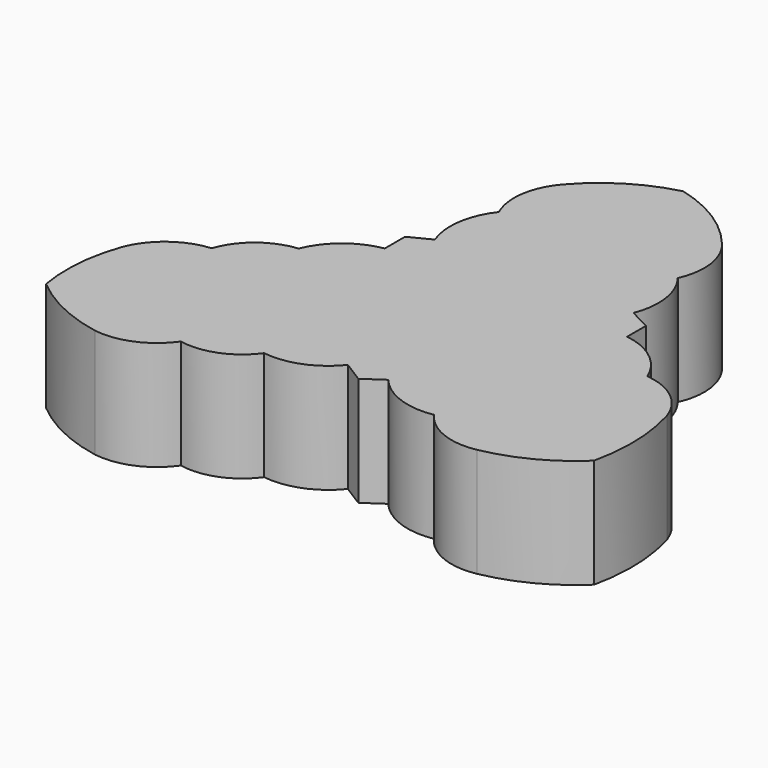
from build123d import *

# Parameters (mm, degrees)
F1_DEPTH = 11.1125


# Not quite as in the source:
# - a length typed as a fraction of an inch, garbled in the dataset ("3 / 203.2 mm" for 3/8 in), is restored


with BuildPart() as f1:
    # F0 (on Top) → F1 (new body)
    with BuildSketch(Plane.XY):
        with BuildLine():
            ThreePointArc((0, 27.0671695471), (-4.5048536548, 25.1556778504), (-8.2258973271, 21.977417171))
            ThreePointArc((-8.2258973271, 21.977417171), (-9.7181261566, 18.698842434), (-9.2097157612, 15.1327075437))
            ThreePointArc((-9.2097157612, 15.1327075437), (-10.6205392688, 11.8246856933), (-10.2093555033, 8.2519613206))
            Line((-10.2093555033, 8.2519613206), (-12.369341217, 7.1464567445))
            Line((-12.369341217, 7.1464567445), (-12.369341217, 4.6386048198))
            Line((-12.369341217, 4.6386048198), (-12.369341217, 4.5682978211))
            ThreePointArc((-12.369341217, 4.5682978211), (-15.5930977879, 3.1185654947), (-17.7027139134, 0.2823972963))
            ThreePointArc((-17.7027139134, 0.2823972963), (-21.0452825194, -1.0603738309), (-23.1384971151, -3.9919692741))
            ThreePointArc((-23.1384971151, -3.9919692741), (-26.5647165348, -5.2934051439), (-28.80180468, -8.19653302))
            ThreePointArc((-28.80180468, -8.19653302), (-29.7673344436, -12.5572908836), (-29.5614041388, -17.0189104974))
            ThreePointArc((-29.5614041388, -17.0189104974), (-25.7783661022, -19.4669407743), (-21.4921734029, -20.8571857766))
            ThreePointArc((-21.4921734029, -20.8571857766), (-17.8594468391, -20.3713745504), (-15.0192606046, -18.054899429))
            ThreePointArc((-15.0192606046, -18.054899429), (-11.4338171794, -17.7079201351), (-8.5996589687, -15.484556372))
            ThreePointArc((-8.5996589687, -15.484556372), (-5.0294162563, -15.0523544446), (-2.1409380715, -12.9098966718))
            Line((-2.1409380715, -12.9098966718), (0, -14.2561570176))
            Line((0, -14.2561570176), (1.9696742658, -12.9098966718))
            ThreePointArc((1.9696742658, -12.9098966718), (4.9392756736, -15.0084468105), (8.560301624, -15.3410370587))
            ThreePointArc((8.560301624, -15.3410370587), (11.3944598347, -17.5644008218), (14.9799032599, -17.9113801157))
            ThreePointArc((14.9799032599, -17.9113801157), (19.5156578324, -16.3470620723), (23.423301056, -13.563092798))
            ThreePointArc((23.423301056, -13.563092798), (23.8861103651, -8.6849198531), (23.0991397704, -3.8484499608))
            ThreePointArc((23.0991397704, -3.8484499608), (21.0059251747, -0.9168545176), (17.6633565687, 0.4259166096))
            ThreePointArc((17.6633565687, 0.4259166096), (15.4847616458, 3.3168082822), (12.1560195839, 4.739132713))
            Line((12.1560195839, 4.739132713), (12.1560195839, 7.1464567445))
            Line((12.1560195839, 7.1464567445), (9.9960338703, 8.2519613206))
            ThreePointArc((9.9960338703, 8.2519613206), (10.4072176357, 11.8246856933), (8.9963941282, 15.1327075437))
            ThreePointArc((8.9963941282, 15.1327075437), (9.5048045235, 18.698842434), (8.012575694, 21.977417171))
            ThreePointArc((8.012575694, 21.977417171), (4.4155385291, 25.1665589), (0, 27.0671695471))
        make_face()
    extrude(amount=F1_DEPTH)


solid = f1.part
